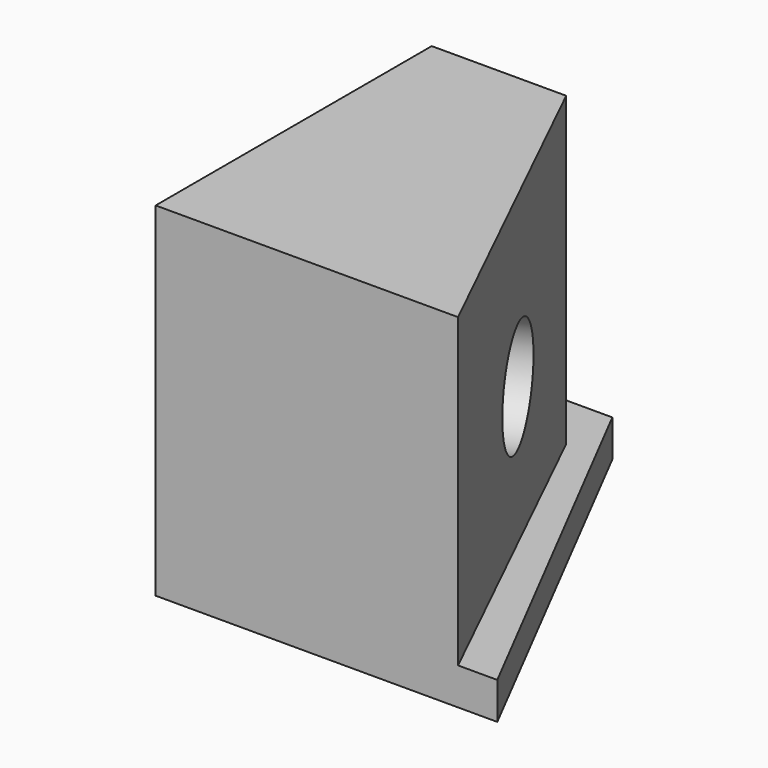
from build123d import *

# Parameters (mm, degrees)
F0_W     = 22.1668612212
F0_H     = 66.4054453373
F1_DEPTH = 6.096
F3_DEPTH = 50.546
F4_R     = 9.1249243662
F5_DEPTH = 27.178


with BuildPart() as f1:
    # F0 (on Top) → F1 (new body)
    with BuildSketch(Plane.XY):
        Polygon((0, 66.4054453373), (0, 0), (34.1540910304, 0), align=None)
        with Locations((-11.0834306106, 33.2027226686)):
            Rectangle(F0_W, F0_H)
    extrude(amount=F1_DEPTH)

    # F2 (on face) → F3 (join)
    with BuildSketch(Plane.XY.offset(6.096)):
        Polygon((0, 56.8917728961), (-22.1668612212, 56.8917728961), (-22.1668612212, 0), (27.6847910136, 0), align=None)
    extrude(amount=F3_DEPTH)

    # F4 (on face) → F5 (cut)
    with BuildSketch(Plane(origin=(22.3841916607, 10.892641178, 0), x_dir=(-0.4375642832, 0.8991871318, 0), z_dir=(0.8991871318, 0.4375642832, 0))):
        with Locations((22.9144543409, 28.7781264633)):
            Circle(F4_R)
    extrude(amount=-F5_DEPTH, mode=Mode.SUBTRACT)


solid = f1.part
